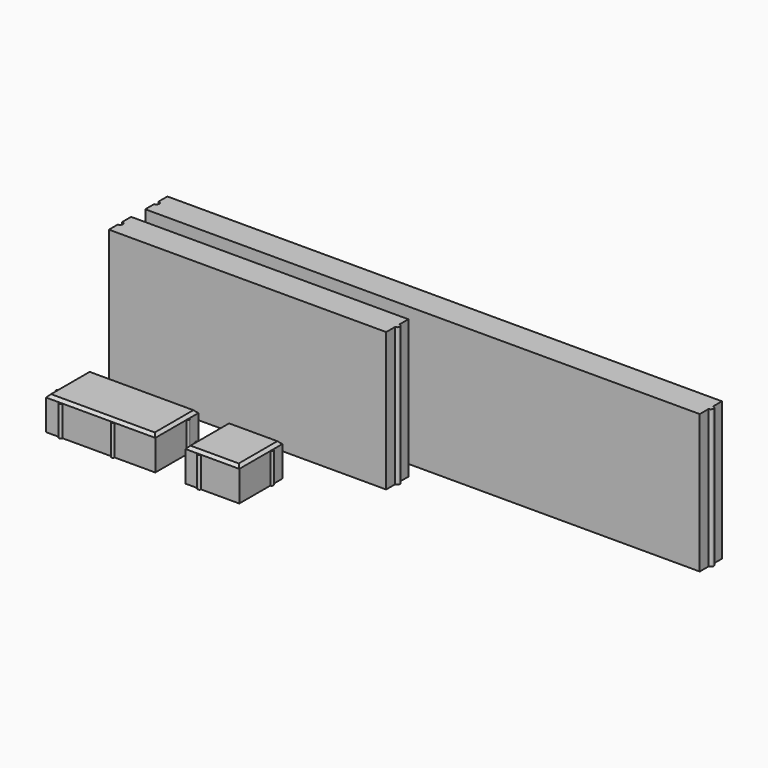
from build123d import *

# Parameters (mm, degrees)
F1_DEPTH = 250
F3_DEPTH = 55
F5_DEPTH = 5
F6_SIZE  = 4.99999
F8_DEPTH = 5
F9_SIZE  = 4.99999


# Not quite as in the source:
# - a fillet or chamfer is up to 0.001 mm smaller than in the source, because OpenCascade refuses the exact size
# - a feature names something its author has since deleted; it is built from what else it names


with BuildPart() as f1:
    # F0 (on Top) → F1 (new body)
    with BuildSketch(Plane.XY):
        with BuildLine():
            Line((-547.6627070457, 65.3239125144), (-547.6627070457, 45.3239125144))
            Line((-547.6627070457, 45.3239125144), (452.3372929543, 45.3239125144))
            Line((452.3372929543, 45.3239125144), (452.3372929543, 65.4239125144))
            ThreePointArc((452.3372929543, 65.4239125144), (457.2372929543, 70.3239125144), (452.3372929543, 75.2239125144))
            Line((452.3372929543, 75.2239125144), (452.3372929543, 95.3239125144))
            Line((452.3372929543, 95.3239125144), (-547.6627070457, 95.3239125144))
            Line((-547.6627070457, 95.3239125144), (-547.6627070457, 75.3239125144))
            ThreePointArc((-547.6627070457, 75.3239125144), (-542.6627070457, 70.3239125144), (-547.6627070457, 65.3239125144))
        make_face()
    extrude(amount=F1_DEPTH)


with BuildPart() as f1b:
    # F0 (on Top) → F1, piece 2 (new body)
    with BuildSketch(Plane.XY):
        with BuildLine():
            Line((-548.7702705837, -15.180903133), (-548.7702705837, -35.180903133))
            Line((-548.7702705837, -35.180903133), (-48.7702705837, -35.180903133))
            Line((-48.7702705837, -35.180903133), (-48.7702705837, -15.080903133))
            ThreePointArc((-48.7702705837, -15.080903133), (-43.8702705837, -10.180903133), (-48.7702705837, -5.280903133))
            Line((-48.7702705837, -5.280903133), (-48.7702705837, 14.819096867))
            Line((-48.7702705837, 14.819096867), (-548.7702705837, 14.819096867))
            Line((-548.7702705837, 14.819096867), (-548.7702705837, -5.180903133))
            ThreePointArc((-548.7702705837, -5.180903133), (-543.7702705837, -10.180903133), (-548.7702705837, -15.180903133))
        make_face()
    extrude(amount=F1_DEPTH)


with BuildPart() as f3:
    # F2 (on Top) → F3 (new body)
    with BuildSketch(Plane.XY):
        with BuildLine():
            Line((-532.024698019, -197.8010260633), (-508.524698019, -197.8010260633))
            ThreePointArc((-508.524698019, -197.8010260633), (-505.524698019, -200.8010260633), (-502.524698019, -197.8010260633))
            Line((-502.524698019, -197.8010260633), (-414.524698019, -197.8010260633))
            ThreePointArc((-414.524698019, -197.8010260633), (-411.524698019, -200.8010260633), (-408.524698019, -197.8010260633))
            Line((-408.524698019, -197.8010260633), (-335.024698019, -197.8010260633))
            Line((-335.024698019, -197.8010260633), (-335.024698019, -127.8537809849))
            ThreePointArc((-335.024698019, -127.8537809849), (-332.024698019, -124.8537809849), (-335.024698019, -121.8537809849))
            Line((-335.024698019, -121.8537809849), (-335.024698019, -100.8010260633))
            Line((-335.024698019, -100.8010260633), (-358.524698019, -100.8010260633))
            ThreePointArc((-358.524698019, -100.8010260633), (-361.524698019, -97.8010260633), (-364.524698019, -100.8010260633))
            Line((-364.524698019, -100.8010260633), (-452.524698019, -100.8010260633))
            ThreePointArc((-452.524698019, -100.8010260633), (-455.524698019, -97.8010260633), (-458.524698019, -100.8010260633))
            Line((-458.524698019, -100.8010260633), (-532.024698019, -100.8010260633))
            Line((-532.024698019, -100.8010260633), (-532.024698019, -168.3010260633))
            ThreePointArc((-532.024698019, -168.3010260633), (-535.024698019, -171.3010260633), (-532.024698019, -174.3010260633))
            Line((-532.024698019, -174.3010260633), (-532.024698019, -197.8010260633))
        make_face()
    extrude(amount=F3_DEPTH)

    # F4 (on face) → F5 (join)
    with BuildSketch(Plane.XY.offset(55)):
        Polygon((-532.024698019, -100.8010260633), (-532.024698019, -168.3010260633), (-532.024698019, -174.3010260633), (-532.024698019, -197.8010260633), (-508.524698019, -197.8010260633), (-502.524698019, -197.8010260633), (-414.524698019, -197.8010260633), (-408.524698019, -197.8010260633), (-335.024698019, -197.8010260633), (-335.024698019, -127.8537809849), (-335.024698019, -121.8537809849), (-335.024698019, -100.8010260633), (-358.524698019, -100.8010260633), (-364.524698019, -100.8010260633), (-452.524698019, -100.8010260633), (-458.524698019, -100.8010260633), align=None)
    extrude(amount=F5_DEPTH)

    # F6 (size 5 in the source; OpenCascade refuses exactly that, so slightly less here)
    f6_edges = [f3.edges().sort_by_distance(p)[0] for p in [
        (-433.524698, -100.801026, 60),
        (-532.024698, -149.301026, 60),
        (-433.524698, -197.801026, 60),
        (-335.024698, -149.301026, 60),
    ]]
    chamfer(f6_edges, length=F6_SIZE)


with BuildPart() as f3b:
    # F2 (on Top) → F3, piece 2 (new body)
    with BuildSketch(Plane.XY):
        Polygon((-280.5922329426, -174.3010260633), (-280.5922329426, -197.8010260633), (-258.5922329426, -197.8010260633), (-252.5922329426, -197.8010260633), (-183.5922329426, -197.8010260633), (-183.5922329426, -127.8537809849), (-183.5922329426, -121.8537809849), (-183.5922329426, -100.8010260633), (-205.5922329426, -100.8010260633), (-211.5922329426, -100.8010260633), (-280.5922329426, -100.8010260633), (-280.5922329426, -168.3010260633), align=None)
        with BuildLine():
            ThreePointArc((-280.5922329426, -168.3010260633), (-283.5922329426, -171.3010260633), (-280.5922329426, -174.3010260633))
            Line((-280.5922329426, -174.3010260633), (-280.5922329426, -168.3010260633))
        make_face()
        with BuildLine():
            Line((-252.5922329426, -197.8010260633), (-258.5922329426, -197.8010260633))
            ThreePointArc((-258.5922329426, -197.8010260633), (-255.5922329426, -200.8010260633), (-252.5922329426, -197.8010260633))
        make_face()
        with BuildLine():
            Line((-183.5922329426, -121.8537809849), (-183.5922329426, -127.8537809849))
            ThreePointArc((-183.5922329426, -127.8537809849), (-180.5922329426, -124.8537809849), (-183.5922329426, -121.8537809849))
        make_face()
        with BuildLine():
            ThreePointArc((-205.5922329426, -100.8010260633), (-208.5922329426, -97.8010260633), (-211.5922329426, -100.8010260633))
            Line((-211.5922329426, -100.8010260633), (-205.5922329426, -100.8010260633))
        make_face()
    extrude(amount=F3_DEPTH)

    # F7 (on face) → F8 (join)
    with BuildSketch(Plane.XY.offset(55)):
        Polygon((-280.5922329426, -168.3010260633), (-280.5922329426, -174.3010260633), (-280.5922329426, -197.8010260633), (-258.5922329426, -197.8010260633), (-252.5922329426, -197.8010260633), (-183.5922329426, -197.8010260633), (-183.5922329426, -127.8537809849), (-183.5922329426, -121.8537809849), (-183.5922329426, -100.8010260633), (-205.5922329426, -100.8010260633), (-211.5922329426, -100.8010260633), (-280.5922329426, -100.8010260633), align=None)
    extrude(amount=F8_DEPTH)

    # F9 (size 5 in the source; OpenCascade refuses exactly that, so slightly less here)
    f9_edges = [f3b.edges().sort_by_distance(p)[0] for p in [
        (-232.092233, -197.801026, 60),
        (-183.592233, -149.301026, 60),
        (-232.092233, -100.801026, 60),
        (-280.592233, -149.301026, 60),
    ]]
    chamfer(f9_edges, length=F9_SIZE)


solid = Compound([f1.part, f1b.part, f3.part, f3b.part])
